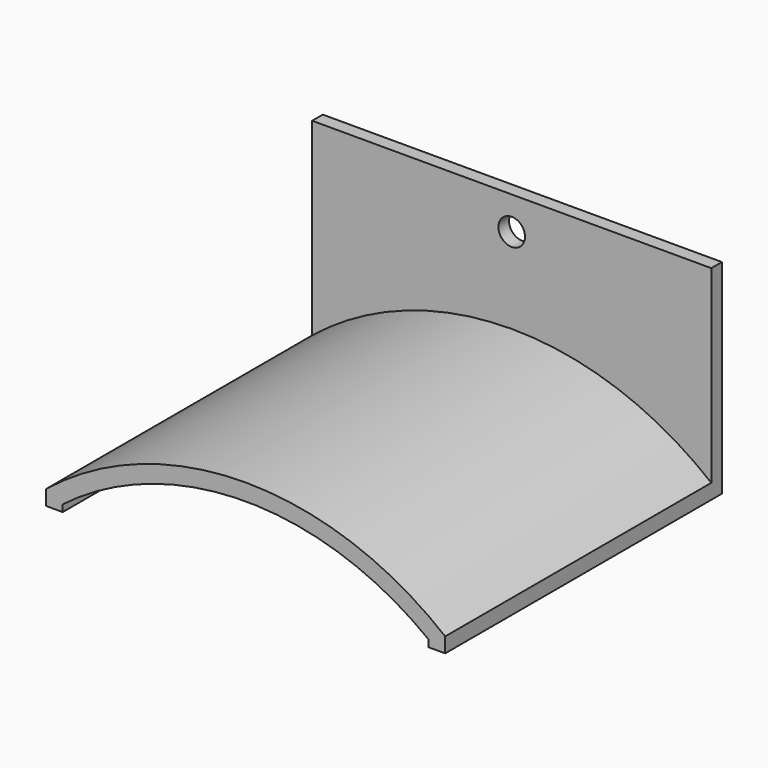
from build123d import *

# Parameters (mm, degrees)
F0_W     = 60
F0_H     = 50
F1_DEPTH = 25
F3_DEPTH = 50.001
F4_W     = 60
F4_H     = 30.659744516
F5_DEPTH = 2
F6_R     = 2
F7_DEPTH = 2.001
F8_T     = -2.5
F9_DEPTH = 25


# Not quite as in the source:
# - a feature of the source that left no trace in its solid (it failed there, or was rolled back) is left out


with BuildPart() as f1:
    # F0 (on Top) → F1 (new body)
    with BuildSketch(Plane.XY):
        Rectangle(F0_W, F0_H)
    extrude(amount=F1_DEPTH)

    # F2 (on face) → F3 (cut, through all)
    with BuildSketch(Plane.XZ.offset(25)):
        with BuildLine():
            ThreePointArc((-30, 2.2523000371), (0, 12.8664154965), (30, 2.2523000371))
            Line((30, 2.2523000371), (30, 25))
            Line((30, 25), (-30, 25))
            Line((-30, 25), (-30, 2.2523000371))
        make_face()
    extrude(amount=-F3_DEPTH, mode=Mode.SUBTRACT)

    # F4 (on face) → F5 (join)
    with BuildSketch(Plane(origin=(0, 25, 0), x_dir=(-1, 0, 0), z_dir=(0, 1, 0))):
        with Locations((0, 15.329872258)):
            Rectangle(F4_W, F4_H)
    extrude(amount=F5_DEPTH)

    # F6 (on face) → F7 (cut, through all)
    with BuildSketch(Plane.XZ.offset(-25)):
        with Locations((0, 25.7051046938)):
            Circle(F6_R)
    extrude(amount=-F7_DEPTH, mode=Mode.SUBTRACT)

    # F8
    f8_openings = [f1.faces().sort_by_distance(p)[0] for p in [
        (0, 1, 0),
    ]]
    offset(amount=F8_T, openings=f8_openings)

    # F9 (cut): a face of the model
    f9_faces = [f1.faces().sort_by_distance(p)[0] for p in [
        (0, -22.5, 4.2031942767),
    ]]
    extrude(f9_faces, amount=-F9_DEPTH, mode=Mode.SUBTRACT)


solid = f1.part
